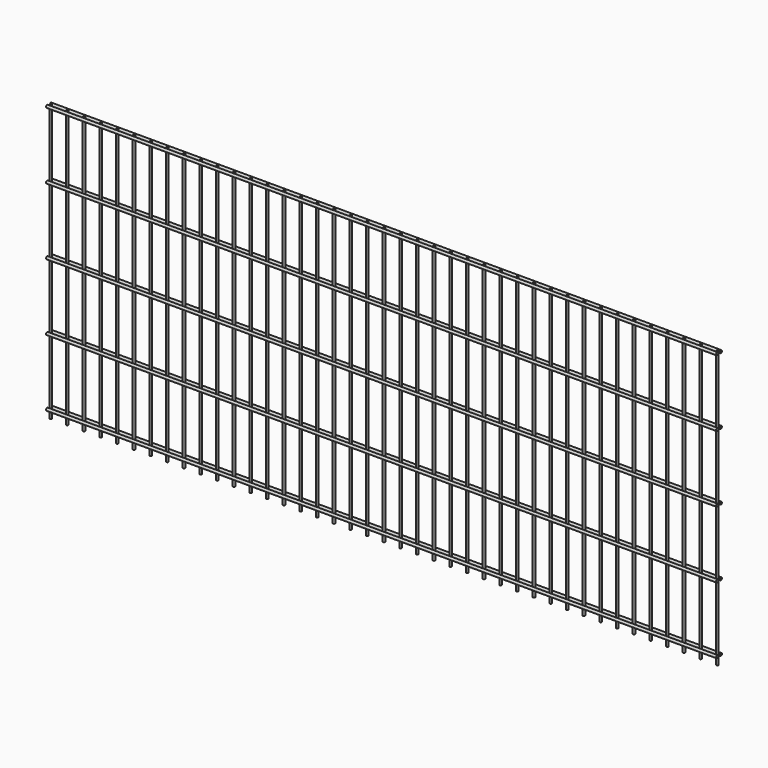
from build123d import *

# Parameters (mm, degrees)
F0_R     = 3
F1_DEPTH = 830
F2_R     = 4
F3_DEPTH = 1005


with BuildPart() as f1:
    # F0 (on Top) → F1 (new body)
    with BuildSketch(Plane.XY):
        with Locations((750, 0)):
            Circle(F0_R)
    extrude(amount=-F1_DEPTH)


with BuildPart() as f1b:
    # F0 (on Top) → F1, piece 2 (new body)
    with BuildSketch(Plane.XY):
        with Locations((-550, 0)):
            Circle(F0_R)
    extrude(amount=-F1_DEPTH)


with BuildPart() as f1c:
    # F0 (on Top) → F1, piece 3 (new body)
    with BuildSketch(Plane.XY):
        with Locations((950, 0)):
            Circle(F0_R)
    extrude(amount=-F1_DEPTH)


with BuildPart() as f1d:
    # F0 (on Top) → F1, piece 4 (new body)
    with BuildSketch(Plane.XY):
        with Locations((450, 0)):
            Circle(F0_R)
    extrude(amount=-F1_DEPTH)


with BuildPart() as f1e:
    # F0 (on Top) → F1, piece 5 (new body)
    with BuildSketch(Plane.XY):
        with Locations((-800, 0)):
            Circle(F0_R)
    extrude(amount=-F1_DEPTH)


with BuildPart() as f1f:
    # F0 (on Top) → F1, piece 6 (new body)
    with BuildSketch(Plane.XY):
        with Locations((-900, 0)):
            Circle(F0_R)
    extrude(amount=-F1_DEPTH)


with BuildPart() as f1g:
    # F0 (on Top) → F1, piece 7 (new body)
    with BuildSketch(Plane.XY):
        with Locations((350, 0)):
            Circle(F0_R)
    extrude(amount=-F1_DEPTH)


with BuildPart() as f1h:
    # F0 (on Top) → F1, piece 8 (new body)
    with BuildSketch(Plane.XY):
        with Locations((-700, 0)):
            Circle(F0_R)
    extrude(amount=-F1_DEPTH)


with BuildPart() as f1i:
    # F0 (on Top) → F1, piece 9 (new body)
    with BuildSketch(Plane.XY):
        with Locations((1000, 0)):
            Circle(F0_R)
    extrude(amount=-F1_DEPTH)


with BuildPart() as f1j:
    # F0 (on Top) → F1, piece 10 (new body)
    with BuildSketch(Plane.XY):
        with Locations((600, 0)):
            Circle(F0_R)
    extrude(amount=-F1_DEPTH)


with BuildPart() as f1k:
    # F0 (on Top) → F1, piece 11 (new body)
    with BuildSketch(Plane.XY):
        with Locations((700, 0)):
            Circle(F0_R)
    extrude(amount=-F1_DEPTH)


with BuildPart() as f1l:
    # F0 (on Top) → F1, piece 12 (new body)
    with BuildSketch(Plane.XY):
        with Locations((650, 0)):
            Circle(F0_R)
    extrude(amount=-F1_DEPTH)


with BuildPart() as f1m:
    # F0 (on Top) → F1, piece 13 (new body)
    with BuildSketch(Plane.XY):
        with Locations((-650, 0)):
            Circle(F0_R)
    extrude(amount=-F1_DEPTH)


with BuildPart() as f1n:
    # F0 (on Top) → F1, piece 14 (new body)
    with BuildSketch(Plane.XY):
        with Locations((850, 0)):
            Circle(F0_R)
    extrude(amount=-F1_DEPTH)


with BuildPart() as f1o:
    # F0 (on Top) → F1, piece 15 (new body)
    with BuildSketch(Plane.XY):
        with Locations((-300, 0)):
            Circle(F0_R)
    extrude(amount=-F1_DEPTH)


with BuildPart() as f1p:
    # F0 (on Top) → F1, piece 16 (new body)
    with BuildSketch(Plane.XY):
        with Locations((-250, 0)):
            Circle(F0_R)
    extrude(amount=-F1_DEPTH)


with BuildPart() as f1q:
    # F0 (on Top) → F1, piece 17 (new body)
    with BuildSketch(Plane.XY):
        with Locations((-350, 0)):
            Circle(F0_R)
    extrude(amount=-F1_DEPTH)


with BuildPart() as f1r:
    # F0 (on Top) → F1, piece 18 (new body)
    with BuildSketch(Plane.XY):
        with Locations((-400, 0)):
            Circle(F0_R)
    extrude(amount=-F1_DEPTH)


with BuildPart() as f1s:
    # F0 (on Top) → F1, piece 19 (new body)
    with BuildSketch(Plane.XY):
        with Locations((-500, 0)):
            Circle(F0_R)
    extrude(amount=-F1_DEPTH)


with BuildPart() as f1t:
    # F0 (on Top) → F1, piece 20 (new body)
    with BuildSketch(Plane.XY):
        with Locations((-950, 0)):
            Circle(F0_R)
    extrude(amount=-F1_DEPTH)


with BuildPart() as f1u:
    # F0 (on Top) → F1, piece 21 (new body)
    with BuildSketch(Plane.XY):
        with Locations((-450, 0)):
            Circle(F0_R)
    extrude(amount=-F1_DEPTH)


with BuildPart() as f1v:
    # F0 (on Top) → F1, piece 22 (new body)
    with BuildSketch(Plane.XY):
        with Locations((150, 0)):
            Circle(F0_R)
    extrude(amount=-F1_DEPTH)


with BuildPart() as f1w:
    # F0 (on Top) → F1, piece 23 (new body)
    with BuildSketch(Plane.XY):
        with Locations((50, 0)):
            Circle(F0_R)
    extrude(amount=-F1_DEPTH)


with BuildPart() as f1x:
    # F0 (on Top) → F1, piece 24 (new body)
    with BuildSketch(Plane.XY):
        with Locations((100, 0)):
            Circle(F0_R)
    extrude(amount=-F1_DEPTH)


with BuildPart() as f1y:
    # F0 (on Top) → F1, piece 25 (new body)
    with BuildSketch(Plane.XY):
        Circle(F0_R)
    extrude(amount=-F1_DEPTH)


with BuildPart() as f1z:
    # F0 (on Top) → F1, piece 26 (new body)
    with BuildSketch(Plane.XY):
        with Locations((-50, 0)):
            Circle(F0_R)
    extrude(amount=-F1_DEPTH)


with BuildPart() as f1ba:
    # F0 (on Top) → F1, piece 27 (new body)
    with BuildSketch(Plane.XY):
        with Locations((-150, 0)):
            Circle(F0_R)
    extrude(amount=-F1_DEPTH)


with BuildPart() as f1bb:
    # F0 (on Top) → F1, piece 28 (new body)
    with BuildSketch(Plane.XY):
        with Locations((-100, 0)):
            Circle(F0_R)
    extrude(amount=-F1_DEPTH)


with BuildPart() as f1bc:
    # F0 (on Top) → F1, piece 29 (new body)
    with BuildSketch(Plane.XY):
        with Locations((-1000, 0)):
            Circle(F0_R)
    extrude(amount=-F1_DEPTH)


with BuildPart() as f1bd:
    # F0 (on Top) → F1, piece 30 (new body)
    with BuildSketch(Plane.XY):
        with Locations((300, 0)):
            Circle(F0_R)
    extrude(amount=-F1_DEPTH)


with BuildPart() as f1be:
    # F0 (on Top) → F1, piece 31 (new body)
    with BuildSketch(Plane.XY):
        with Locations((250, 0)):
            Circle(F0_R)
    extrude(amount=-F1_DEPTH)


with BuildPart() as f1bf:
    # F0 (on Top) → F1, piece 32 (new body)
    with BuildSketch(Plane.XY):
        with Locations((-200, 0)):
            Circle(F0_R)
    extrude(amount=-F1_DEPTH)


with BuildPart() as f1bg:
    # F0 (on Top) → F1, piece 33 (new body)
    with BuildSketch(Plane.XY):
        with Locations((900, 0)):
            Circle(F0_R)
    extrude(amount=-F1_DEPTH)


with BuildPart() as f1bh:
    # F0 (on Top) → F1, piece 34 (new body)
    with BuildSketch(Plane.XY):
        with Locations((-750, 0)):
            Circle(F0_R)
    extrude(amount=-F1_DEPTH)


with BuildPart() as f1bi:
    # F0 (on Top) → F1, piece 35 (new body)
    with BuildSketch(Plane.XY):
        with Locations((200, 0)):
            Circle(F0_R)
    extrude(amount=-F1_DEPTH)


with BuildPart() as f1bj:
    # F0 (on Top) → F1, piece 36 (new body)
    with BuildSketch(Plane.XY):
        with Locations((500, 0)):
            Circle(F0_R)
    extrude(amount=-F1_DEPTH)


with BuildPart() as f1bk:
    # F0 (on Top) → F1, piece 37 (new body)
    with BuildSketch(Plane.XY):
        with Locations((550, 0)):
            Circle(F0_R)
    extrude(amount=-F1_DEPTH)


with BuildPart() as f1bl:
    # F0 (on Top) → F1, piece 38 (new body)
    with BuildSketch(Plane.XY):
        with Locations((-600, 0)):
            Circle(F0_R)
    extrude(amount=-F1_DEPTH)


with BuildPart() as f1bm:
    # F0 (on Top) → F1, piece 39 (new body)
    with BuildSketch(Plane.XY):
        with Locations((800, 0)):
            Circle(F0_R)
    extrude(amount=-F1_DEPTH)


with BuildPart() as f1bn:
    # F0 (on Top) → F1, piece 40 (new body)
    with BuildSketch(Plane.XY):
        with Locations((-850, 0)):
            Circle(F0_R)
    extrude(amount=-F1_DEPTH)


with BuildPart() as f1bo:
    # F0 (on Top) → F1, piece 41 (new body)
    with BuildSketch(Plane.XY):
        with Locations((400, 0)):
            Circle(F0_R)
    extrude(amount=-F1_DEPTH)


with BuildPart() as f3:
    # F2 (on Right) → F3 (new body, symmetric)
    with BuildSketch(Plane.YZ):
        with Locations((7, -4)):
            Circle(F2_R)
    extrude(amount=F3_DEPTH, both=True)


with BuildPart() as f3b:
    # F2 (on Right) → F3, piece 2 (new body, symmetric)
    with BuildSketch(Plane.YZ):
        with Locations((-7, -4)):
            Circle(F2_R)
    extrude(amount=F3_DEPTH, both=True)


with BuildPart() as f3c:
    # F2 (on Right) → F3, piece 3 (new body, symmetric)
    with BuildSketch(Plane.YZ):
        with Locations((7, -204)):
            Circle(F2_R)
    extrude(amount=F3_DEPTH, both=True)


with BuildPart() as f3d:
    # F2 (on Right) → F3, piece 4 (new body, symmetric)
    with BuildSketch(Plane.YZ):
        with Locations((-7, -204)):
            Circle(F2_R)
    extrude(amount=F3_DEPTH, both=True)


with BuildPart() as f3e:
    # F2 (on Right) → F3, piece 5 (new body, symmetric)
    with BuildSketch(Plane.YZ):
        with Locations((7, -404)):
            Circle(F2_R)
    extrude(amount=F3_DEPTH, both=True)


with BuildPart() as f3f:
    # F2 (on Right) → F3, piece 6 (new body, symmetric)
    with BuildSketch(Plane.YZ):
        with Locations((-7, -404)):
            Circle(F2_R)
    extrude(amount=F3_DEPTH, both=True)


with BuildPart() as f3g:
    # F2 (on Right) → F3, piece 7 (new body, symmetric)
    with BuildSketch(Plane.YZ):
        with Locations((7, -604)):
            Circle(F2_R)
    extrude(amount=F3_DEPTH, both=True)


with BuildPart() as f3h:
    # F2 (on Right) → F3, piece 8 (new body, symmetric)
    with BuildSketch(Plane.YZ):
        with Locations((-7, -604)):
            Circle(F2_R)
    extrude(amount=F3_DEPTH, both=True)


with BuildPart() as f3i:
    # F2 (on Right) → F3, piece 9 (new body, symmetric)
    with BuildSketch(Plane.YZ):
        with Locations((7, -804)):
            Circle(F2_R)
    extrude(amount=F3_DEPTH, both=True)


with BuildPart() as f3j:
    # F2 (on Right) → F3, piece 10 (new body, symmetric)
    with BuildSketch(Plane.YZ):
        with Locations((-7, -804)):
            Circle(F2_R)
    extrude(amount=F3_DEPTH, both=True)


solid = Compound([f1.part, f1b.part, f1c.part, f1d.part, f1e.part, f1f.part, f1g.part, f1h.part, f1i.part, f1j.part, f1k.part, f1l.part, f1m.part, f1n.part, f1o.part, f1p.part, f1q.part, f1r.part, f1s.part, f1t.part, f1u.part, f1v.part, f1w.part, f1x.part, f1y.part, f1z.part, f1ba.part, f1bb.part, f1bc.part, f1bd.part, f1be.part, f1bf.part, f1bg.part, f1bh.part, f1bi.part, f1bj.part, f1bk.part, f1bl.part, f1bm.part, f1bn.part, f1bo.part, f3.part, f3b.part, f3c.part, f3d.part, f3e.part, f3f.part, f3g.part, f3h.part, f3i.part, f3j.part])
